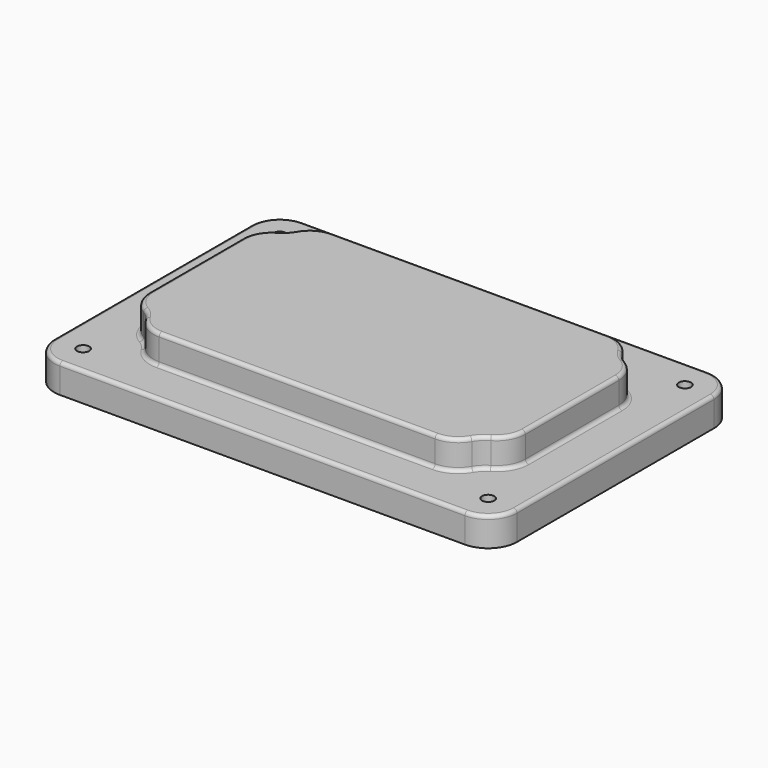
from build123d import *

# Parameters (mm, degrees)
F1_DEPTH  = 6.35
F2_W      = 82.55
F2_H      = 47.625
F3_DEPTH  = 6.35
F4_R      = 6.35
F5_DEPTH  = 6.35
F6_R      = 6.35
F7_DEPTH  = 6.35
F8_R      = 6.35
F9_T      = -3.175
F10_R     = 6.35
F11_DEPTH = 3.175
F12_R     = 0.78739
F14_D     = 2.7051


# Not quite as in the source:
# - a fillet or chamfer is up to 0.001 mm smaller than in the source, because OpenCascade refuses the exact size


with BuildPart() as f1:
    # F0 (on Top) → F1 (new body)
    with BuildSketch(Plane.XY):
        with BuildLine():
            Line((44.45, 33.3375), (-44.45, 33.3375))
            ThreePointArc((-44.45, 33.3375), (-48.9401280605, 31.4776280605), (-50.8, 26.9875))
            Line((-50.8, 26.9875), (-50.8, -26.9875))
            ThreePointArc((-50.8, -26.9875), (-48.9401280605, -31.4776280605), (-44.45, -33.3375))
            Line((-44.45, -33.3375), (44.45, -33.3375))
            ThreePointArc((44.45, -33.3375), (48.9401280605, -31.4776280605), (50.8, -26.9875))
            Line((50.8, -26.9875), (50.8, 26.9875))
            ThreePointArc((50.8, 26.9875), (48.9401280605, 31.4776280605), (44.45, 33.3375))
        make_face()
    extrude(amount=F1_DEPTH)

    # F2 (on face) → F3 (join)
    with BuildSketch(Plane.XY.offset(6.35)):
        Rectangle(F2_W, F2_H)
    extrude(amount=F3_DEPTH)

    # F4 (on face) → F5 (cut, through all)
    with BuildSketch(Plane.XY.offset(12.7)):
        with Locations((41.275, 23.8125)):
            Circle(F4_R)
        with Locations((41.275, -23.8125)):
            Circle(F4_R)
    extrude(amount=-F5_DEPTH, mode=Mode.SUBTRACT)

    # F6 (on face) → F7 (cut, through all)
    with BuildSketch(Plane.XY.offset(12.7)):
        with Locations((-41.275, 23.8125)):
            Circle(F6_R)
        with Locations((-41.275, -23.8125)):
            Circle(F6_R)
    extrude(amount=-F7_DEPTH, mode=Mode.SUBTRACT)

    # F8
    f8_edges = [f1.edges().sort_by_distance(p)[0] for p in [
        (-34.925, -23.8125, 9.525),
        (-41.275, -17.4625, 9.525),
        (-41.275, 17.4625, 9.525),
        (-34.925, 23.8125, 9.525),
        (34.925, 23.8125, 9.525),
        (41.275, 17.4625, 9.525),
        (41.275, -17.4625, 9.525),
        (34.925, -23.8125, 9.525),
    ]]
    fillet(f8_edges, radius=F8_R)

    # F9
    f9_openings = [f1.faces().sort_by_distance(p)[0] for p in [
        (0, 0, 0),
    ]]
    offset(amount=F9_T, openings=f9_openings, kind=Kind.INTERSECTION)

    # F10 (on face) → F11 (join, through all)
    with BuildSketch(Plane(origin=(0, 0, 0), x_dir=(1, 0, 0), z_dir=(0, 0, -1))):
        with Locations((44.45, 26.9875)):
            Circle(F10_R)
        with Locations((44.45, -26.9875)):
            Circle(F10_R)
        with Locations((-44.45, -26.9875)):
            Circle(F10_R)
        with Locations((-44.45, 26.9875)):
            Circle(F10_R)
    extrude(amount=-F11_DEPTH)

    # F12 (radius 0.7874 in the source; OpenCascade refuses exactly that, so slightly less here)
    f12_edges = [f1.edges().sort_by_distance(p)[0] for p in [
        (-47.625, 0, 3.175),
        (-39.959872, -22.497372, 3.175),
        (0, -30.1625, 3.175),
        (39.959872, -22.497372, 3.175),
        (47.625, 0, 3.175),
        (39.959872, 22.497372, 3.175),
        (0, 30.1625, 3.175),
        (-39.959872, 22.497372, 3.175),
        (0, 20.6375, 3.175),
        (31.863977, 20.212131, 3.175),
        (34.539808, 17.077308, 3.175),
        (37.674631, 14.401477, 3.175),
        (38.1, 0, 3.175),
        (37.674631, -14.401477, 3.175),
        (34.539808, -17.077308, 3.175),
        (31.863977, -20.212131, 3.175),
        (0, -20.6375, 3.175),
        (-31.863977, -20.212131, 3.175),
        (-34.539808, -17.077308, 3.175),
        (-37.674631, -14.401477, 3.175),
        (-38.1, 0, 3.175),
        (-37.674631, 14.401477, 3.175),
        (-34.539808, 17.077308, 3.175),
        (-31.863977, 20.212131, 3.175),
        (0, 20.6375, 9.525),
        (-31.863977, 20.212131, 9.525),
        (-34.539808, 17.077308, 9.525),
        (-37.674631, 14.401477, 9.525),
        (-38.1, 0, 9.525),
        (-37.674631, -14.401477, 9.525),
        (-34.539808, -17.077308, 9.525),
        (-31.863977, -20.212131, 9.525),
        (0, -20.6375, 9.525),
        (31.863977, -20.212131, 9.525),
        (34.539808, -17.077308, 9.525),
        (37.674631, -14.401477, 9.525),
        (38.1, 0, 9.525),
        (37.674631, 14.401477, 9.525),
        (34.539808, 17.077308, 9.525),
        (31.863977, 20.212131, 9.525),
        (-47.625, 0, 0),
        (0, 30.1625, 0),
        (47.625, 0, 0),
        (39.959872, 22.497372, 0),
        (39.959872, -22.497372, 0),
        (0, -30.1625, 0),
        (-39.959872, -22.497372, 0),
        (36.784872, 19.322372, 12.7),
        (33.451477, 22.961761, 12.7),
        (40.424261, 15.988977, 12.7),
        (0, 23.8125, 12.7),
        (41.275, 0, 12.7),
        (-33.451477, 22.961761, 12.7),
        (40.424261, -15.988977, 12.7),
        (-36.784872, 19.322372, 12.7),
        (36.784872, -19.322372, 12.7),
        (-40.424261, 15.988977, 12.7),
        (33.451477, -22.961761, 12.7),
        (-41.275, 0, 12.7),
        (0, -23.8125, 12.7),
        (-40.424261, -15.988977, 12.7),
        (-33.451477, -22.961761, 12.7),
        (-36.784872, -19.322372, 12.7),
        (0, 23.8125, 6.35),
        (33.451477, 22.961761, 6.35),
        (-33.451477, 22.961761, 6.35),
        (36.784872, 19.322372, 6.35),
        (-36.784872, 19.322372, 6.35),
        (40.424261, 15.988977, 6.35),
        (-40.424261, 15.988977, 6.35),
        (41.275, 0, 6.35),
        (-41.275, 0, 6.35),
        (40.424261, -15.988977, 6.35),
        (-40.424261, -15.988977, 6.35),
        (36.784872, -19.322372, 6.35),
        (-36.784872, -19.322372, 6.35),
        (33.451477, -22.961761, 6.35),
        (-33.451477, -22.961761, 6.35),
        (0, -23.8125, 6.35),
        (0, 33.3375, 6.35),
        (-48.940128, 31.477628, 6.35),
        (-50.8, 0, 6.35),
        (-48.940128, -31.477628, 6.35),
        (0, -33.3375, 6.35),
        (48.940128, -31.477628, 6.35),
        (50.8, 0, 6.35),
        (48.940128, 31.477628, 6.35),
        (-39.959872, 22.497372, 0),
    ]]
    fillet(f12_edges, radius=F12_R)

    # F14 (through all)
    with Locations(Plane(origin=(0, 0, 0), x_dir=(1, 0, 0), z_dir=(0, 0, -1))):
        with Locations((-44.45, 26.9875), (-44.45, -26.9875), (44.45, -26.9875), (44.45, 26.9875)):
            Hole(F14_D / 2)


solid = f1.part
